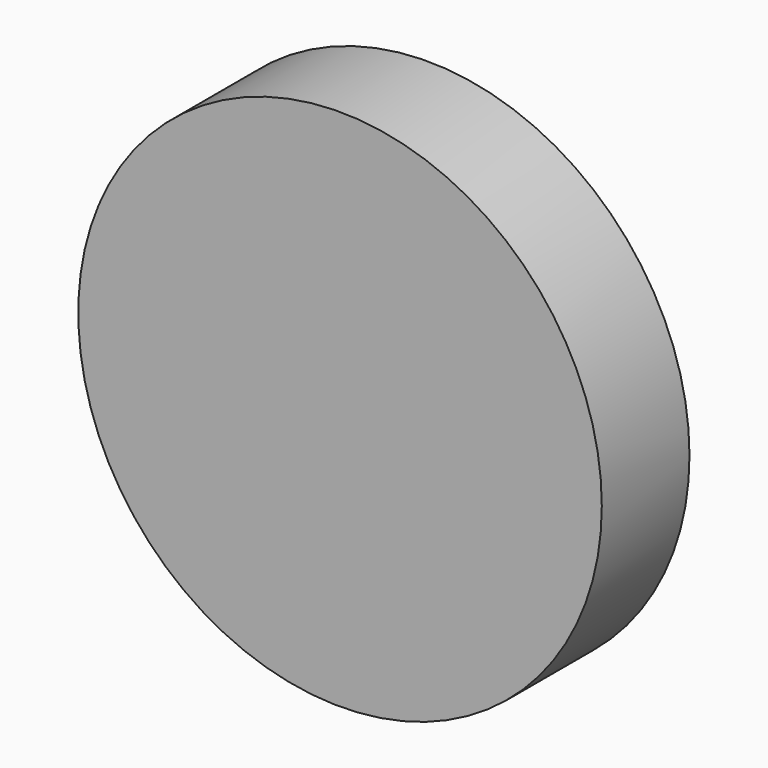
from build123d import *

# Parameters (mm, degrees)
F1_R     = 50.8
F2_DEPTH = 21.2725


# Not quite as in the source:
# - a length typed as a fraction of an inch, garbled in the dataset ("3 / 203.2 mm" for 3/8 in), is restored


with BuildPart() as f2:
    # F1 (on Front) → F2 (new body)
    with BuildSketch(Plane.XZ):
        Circle(F1_R)
    extrude(amount=F2_DEPTH)


solid = f2.part
